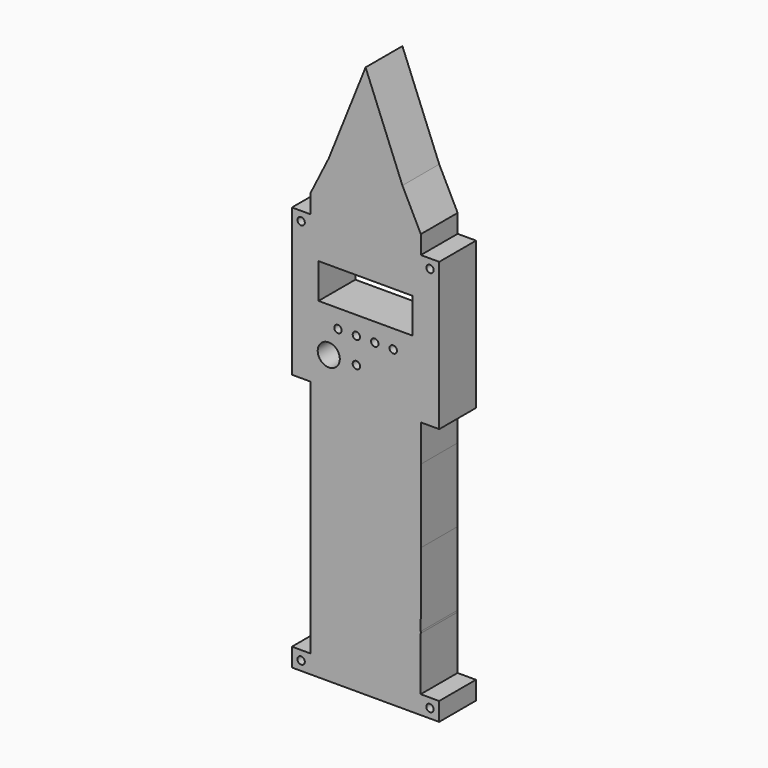
from build123d import *

# Parameters (mm, degrees)
F0_R     = 2
F0_R_2   = 6
F0_W     = 51.13
F0_H     = 19.04
F1_DEPTH = 25


# Not quite as in the source:
# - ends of sketch curves that miss each other by under 0.0002 mm in the source are joined


with BuildPart() as f1:
    # F0 (on Front) → F1 (new body)
    with BuildSketch(Plane.XZ):
        with BuildLine():
            Line((-0.0546134975, 0), (0, 0))
            Line((0, 0), (39.9453865025, 1.14717e-05))
            Line((39.9453865025, 1.14717e-05), (39.9453865025, 10.0000114717))
            Line((39.9453865025, 10.0000114717), (29.9453865025, 10.0000114717))
            Line((29.9453865025, 10.0000114717), (29.9576031817, 39.0801515195))
            ThreePointArc((29.9576031817, 39.0801515195), (24.9768942877, 34.5421678148), (20, 39.0843347471))
            ThreePointArc((20, 39.0843347471), (19.9842488656, 39.3130102593), (19.9789948068, 39.5421673735))
            ThreePointArc((19.9789948068, 39.5421673735), (14.7708428858, 35.0052540588), (10, 40))
            ThreePointArc((10, 40), (5, 35), (0, 40))
            ThreePointArc((0, 40), (-5, 35), (-10, 40))
            ThreePointArc((-10, 40), (-15, 35), (-20, 40))
            ThreePointArc((-20, 40), (-25, 35), (-30, 40))
            Line((-30, 40), (-30, 10))
            Line((-30, 10), (-40, 10))
            Line((-40, 10), (-40, 0))
            Line((-40, 0), (-0.0546134975, 0))
        make_face()
        with Locations((-35, 5)):
            Circle(F0_R, mode=Mode.SUBTRACT)
        with Locations((34.9453865025, 5.0000114717)):
            Circle(F0_R, mode=Mode.SUBTRACT)
        with BuildLine():
            ThreePointArc((20, 39.0843347471), (24.9768942877, 34.5421678148), (29.9576031817, 39.0801515195))
            Line((29.9576031817, 39.0801515195), (29.9579896136, 40))
            Line((29.9579896136, 40), (29.9747937682, 80))
            ThreePointArc((29.9747937682, 80), (24.9873968841, 75.3547848935), (20, 80))
            Line((20, 80), (20, 40))
            Line((20, 40), (20, 39.0843347471))
        make_face()
        with BuildLine():
            Line((29.9579896136, 40), (29.9576031817, 39.0801515195))
            ThreePointArc((29.9576031817, 39.0801515195), (29.9789943656, 39.5400668544), (29.9579896136, 40))
        make_face()
        with BuildLine():
            Line((-30, 80), (-30, 40))
            ThreePointArc((-30, 40), (-25, 35), (-20, 40))
            Line((-20, 40), (-20, 80))
            ThreePointArc((-20, 80), (-25, 75), (-30, 80))
        make_face()
        with BuildLine():
            Line((-30, 120), (-30, 80))
            ThreePointArc((-30, 80), (-25, 75), (-20, 80))
            Line((-20, 80), (-20, 120))
            ThreePointArc((-20, 120), (-25, 115), (-30, 120))
        make_face()
        with BuildLine():
            ThreePointArc((20, 80), (24.9873968841, 75.3547848935), (29.9747937682, 80))
            Line((29.9747937682, 80), (29.9915979227, 120))
            ThreePointArc((29.9915979227, 120), (24.9957989614, 115.2049212963), (20, 120))
            Line((20, 120), (20, 80))
        make_face()
        with BuildLine():
            Line((-30, 140), (-30, 120))
            ThreePointArc((-30, 120), (-25, 115), (-20, 120))
            Line((-20, 120), (-20, 140))
            Line((-20, 140), (-30, 140))
        make_face()
        with BuildLine():
            ThreePointArc((20, 120), (24.9957989614, 115.2049212963), (29.9915979227, 120))
            Line((29.9915979227, 120), (30, 140))
            Line((30, 140), (20, 140))
            Line((20, 140), (20, 120))
        make_face()
        Polygon((-40, 140), (-30, 140), (-20, 140), (-10, 140), (0, 140), (10, 140), (20, 140), (30, 140), (40, 140), (40, 220), (30, 220), (-30, 220), (-40, 220), align=None)
        with Locations((-35, 215)):
            Circle(F0_R, mode=Mode.SUBTRACT)
        with Locations((-20, 156)):
            Circle(F0_R_2, mode=Mode.SUBTRACT)
        with Locations((-15, 170)):
            Circle(F0_R, mode=Mode.SUBTRACT)
        with Locations((-5, 156)):
            Circle(F0_R, mode=Mode.SUBTRACT)
        with Locations((-5, 170)):
            Circle(F0_R, mode=Mode.SUBTRACT)
        with Locations((5, 170)):
            Circle(F0_R, mode=Mode.SUBTRACT)
        with Locations((15, 170)):
            Circle(F0_R, mode=Mode.SUBTRACT)
        with Locations((0, 189.52)):
            Rectangle(F0_W, F0_H, mode=Mode.SUBTRACT)
        with Locations((35, 215)):
            Circle(F0_R, mode=Mode.SUBTRACT)
        Polygon((-30, 230), (-30, 220), (30, 220), (30, 230), (0, 230), align=None)
        Polygon((-20, 250), (-30, 230), (0, 230), (30, 230), (20, 250), (0, 250), align=None)
        Polygon((0, 300), (-20, 250), (0, 250), (20, 250), align=None)
        with BuildLine():
            Line((-20, 120), (-20, 80))
            ThreePointArc((-20, 80), (-15, 75), (-10, 80))
            Line((-10, 80), (-10, 120))
            ThreePointArc((-10, 120), (-15, 115), (-20, 120))
        make_face()
        with BuildLine():
            Line((-10, 120), (-10, 80))
            ThreePointArc((-10, 80), (-5, 75), (0, 80))
            Line((0, 80), (0, 120))
            ThreePointArc((0, 120), (-5, 115), (-10, 120))
        make_face()
        with BuildLine():
            ThreePointArc((0, 80), (5, 75), (10, 80))
            Line((10, 80), (10, 120))
            ThreePointArc((10, 120), (5, 115), (0, 120))
            Line((0, 120), (0, 80))
        make_face()
        with BuildLine():
            ThreePointArc((10, 80), (15, 75), (20, 80))
            Line((20, 80), (20, 120))
            ThreePointArc((20, 120), (15, 115), (10, 120))
            Line((10, 120), (10, 80))
        make_face()
        with BuildLine():
            ThreePointArc((19.9789948068, 39.5421673735), (19.9842488656, 39.7713244878), (20, 40))
            Line((20, 40), (20, 80))
            ThreePointArc((20, 80), (15, 75), (10, 80))
            Line((10, 80), (10, 40))
            ThreePointArc((10, 40), (14.7708428858, 35.0052540588), (19.9789948068, 39.5421673735))
        make_face()
        with BuildLine():
            ThreePointArc((0, 40), (5, 35), (10, 40))
            Line((10, 40), (10, 80))
            ThreePointArc((10, 80), (5, 75), (0, 80))
            Line((0, 80), (0, 40))
        make_face()
        with BuildLine():
            Line((-10, 80), (-10, 40))
            ThreePointArc((-10, 40), (-5, 35), (0, 40))
            Line((0, 40), (0, 80))
            ThreePointArc((0, 80), (-5, 75), (-10, 80))
        make_face()
        with BuildLine():
            Line((-20, 80), (-20, 40))
            ThreePointArc((-20, 40), (-15, 35), (-10, 40))
            Line((-10, 40), (-10, 80))
            ThreePointArc((-10, 80), (-15, 75), (-20, 80))
        make_face()
        with BuildLine():
            Line((-20, 140), (-20, 120))
            ThreePointArc((-20, 120), (-15, 115), (-10, 120))
            Line((-10, 120), (-10, 140))
            Line((-10, 140), (-20, 140))
        make_face()
        with BuildLine():
            Line((-10, 140), (-10, 120))
            ThreePointArc((-10, 120), (-5, 115), (0, 120))
            Line((0, 120), (0, 140))
            Line((0, 140), (-10, 140))
        make_face()
        with BuildLine():
            ThreePointArc((0, 120), (5, 115), (10, 120))
            Line((10, 120), (10, 140))
            Line((10, 140), (0, 140))
            Line((0, 140), (0, 120))
        make_face()
        with BuildLine():
            ThreePointArc((10, 120), (15, 115), (20, 120))
            Line((20, 120), (20, 140))
            Line((20, 140), (10, 140))
            Line((10, 140), (10, 120))
        make_face()
    extrude(amount=F1_DEPTH)


solid = f1.part
